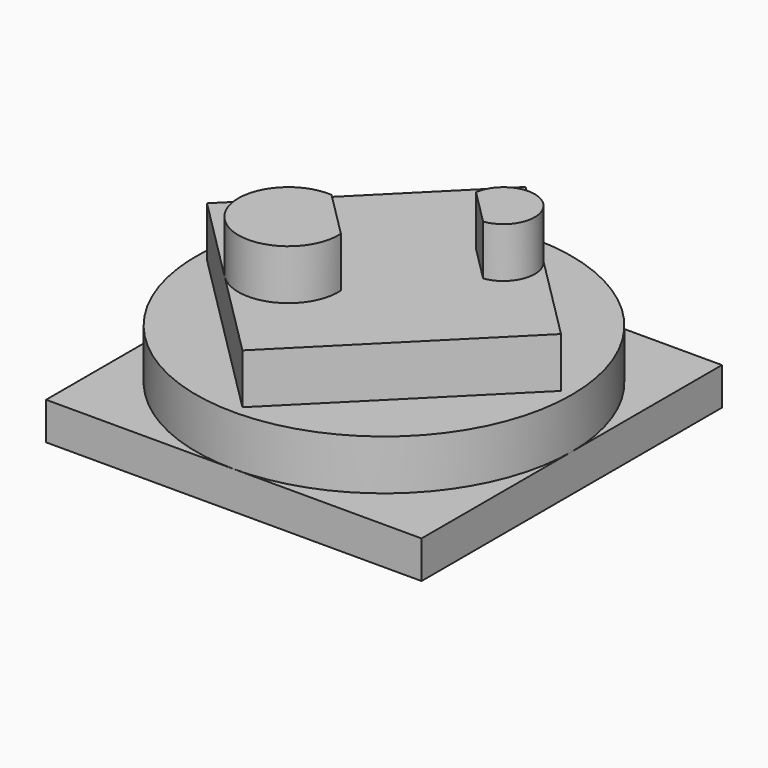
from build123d import *

# Parameters (mm, degrees)
F0_W     = 30
F0_H     = 30
F1_DEPTH = 3
F2_R     = 15
F3_DEPTH = 4
F5_DEPTH = 4
F7_DEPTH = 4


# Not quite as in the source:
# - a feature names something its author has since deleted; it is built from what else it names


with BuildPart() as f1:
    # F0 (on Top) → F1 (new body)
    with BuildSketch(Plane.XY):
        Rectangle(F0_W, F0_H)
    extrude(amount=F1_DEPTH)

    # F2 (on face) → F3 (join)
    with BuildSketch(Plane.XY.offset(3)):
        Circle(F2_R)
    extrude(amount=F3_DEPTH)

    # F4 (on face) → F5 (join)
    with BuildSketch(Plane.XY.offset(7)):
        Polygon((14.1421356237, 0), (0, 14.1421356237), (-14.1421356237, 0), (0, -14.1421356237), align=None)
    extrude(amount=F5_DEPTH)

    # F6 (on face) → F7 (join)
    with BuildSketch(Plane.XY.offset(11)):
        with BuildLine():
            Line((2.8284271247, 5.6568542495), (5.6568542495, 2.8284271247))
            ThreePointArc((5.6568542495, 2.8284271247), (7.0710678119, 7.0710678119), (2.8284271247, 5.6568542495))
        make_face()
        with BuildLine():
            Line((-0.2504916502, -3.9921490369), (-3.9921490369, -0.2504916502))
            ThreePointArc((-3.9921490369, -0.2504916502), (-7.0710678119, -7.0710678119), (-0.2504916502, -3.9921490369))
        make_face()
    extrude(amount=F7_DEPTH)


solid = f1.part
